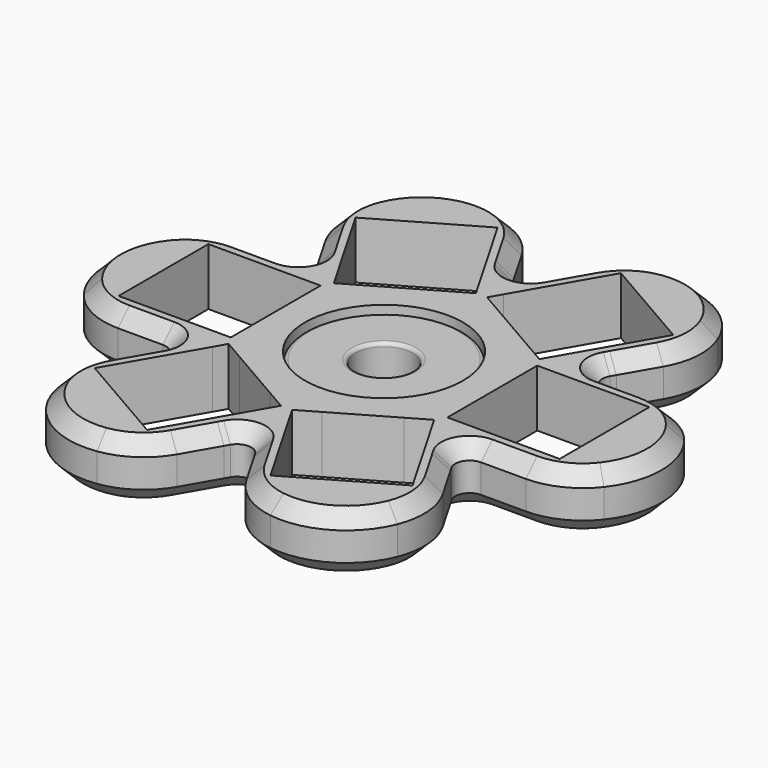
from build123d import *

# Parameters (mm, degrees)
F0_R     = 11
F0_R_2   = 4
F1_DEPTH = 7
F2_R     = 11.05
F3_DEPTH = 8
F4_R     = 2
F5_R     = 10
F6_SIZE  = 2
F7_R     = 0.5


# Not quite as in the source:
# - a feature names something its author has since deleted; it is built from what else it names


with BuildPart() as f1:
    # F0 (on Top) → F1 (new body)
    with BuildSketch(Plane.XY):
        Circle(F0_R)
        Circle(F0_R_2, mode=Mode.SUBTRACT)
    extrude(amount=F1_DEPTH)

    # F7
    f7_edges = [f1.edges().sort_by_distance(p)[0] for p in [
        (-11, 0, 0),
        (-4, 0, 0),
        (-11, 0, 7),
        (-4, 0, 7),
    ]]
    fillet(f7_edges, radius=F7_R)


with BuildPart() as f3:
    # F2 (on face) → F3 (new body)
    with BuildSketch(Plane(origin=(0, 0, 0), x_dir=(1, 0, 0), z_dir=(0, 0, -1))):
        with BuildLine():
            Line((18.7927512621, -10.85), (15.328649647, -10.85))
            Line((15.328649647, -10.85), (22.2232994197, -22.7918837067))
            Line((22.2232994197, -22.7918837067), (8.6267005803, -30.6418837067))
            Line((8.6267005803, -30.6418837067), (1.7320508076, -18.7))
            Line((1.7320508076, -18.7), (0, -21.7))
            Line((0, -21.7), (2.1036243689, -25.343584287))
            Line((2.1036243689, -25.343584287), (6.0286243689, -32.1418837067))
            ThreePointArc((6.0286243689, -32.1418837067), (19.4, -33.6017856668), (24.8213756311, -21.2918837067))
            Line((24.8213756311, -21.2918837067), (20.8963756311, -14.493584287))
            Line((20.8963756311, -14.493584287), (18.7927512621, -10.85))
        make_face()
        with BuildLine():
            Line((15.15, -4.5405697347), (14.6112581801, -3.6074415304))
            ThreePointArc((14.6112581801, -3.6074415304), (13.033682327, -7.525), (10.429765098, -10.85))
            Line((10.429765098, -10.85), (11.5072487379, -10.85))
            Line((11.5072487379, -10.85), (14.3732994197, -9.1952848673))
            Line((14.3732994197, -9.1952848673), (15.328649647, -10.85))
            Line((15.328649647, -10.85), (18.7927512621, -10.85))
            Line((18.7927512621, -10.85), (17.0607004546, -7.85))
            Line((17.0607004546, -7.85), (15.15, -7.85))
            Line((15.15, -7.85), (15.15, -4.5405697347))
        make_face()
        with BuildLine():
            ThreePointArc((14.6112581801, -3.6074415304), (14.9399119075, -1.8170118863), (15.05, 0))
            ThreePointArc((15.05, 0), (14.9399119075, 1.8170118863), (14.6112581801, 3.6074415304))
            ThreePointArc((14.6112581801, 3.6074415304), (13.033682327, 7.525), (10.429765098, 10.85))
            ThreePointArc((10.429765098, 10.85), (7.525, 13.033682327), (4.181493082, 14.4574415304))
            ThreePointArc((4.181493082, 14.4574415304), (0, 15.05), (-4.181493082, 14.4574415304))
            ThreePointArc((-4.181493082, 14.4574415304), (-7.525, 13.033682327), (-10.429765098, 10.85))
            ThreePointArc((-10.429765098, 10.85), (-13.033682327, 7.525), (-14.6112581801, 3.6074415304))
            ThreePointArc((-14.6112581801, 3.6074415304), (-15.05, 0), (-14.6112581801, -3.6074415304))
            ThreePointArc((-14.6112581801, -3.6074415304), (-13.033682327, -7.525), (-10.429765098, -10.85))
            ThreePointArc((-10.429765098, -10.85), (-7.525, -13.033682327), (-4.181493082, -14.4574415304))
            ThreePointArc((-4.181493082, -14.4574415304), (0, -15.05), (4.181493082, -14.4574415304))
            ThreePointArc((4.181493082, -14.4574415304), (7.525, -13.033682327), (10.429765098, -10.85))
            ThreePointArc((10.429765098, -10.85), (13.033682327, -7.525), (14.6112581801, -3.6074415304))
        make_face()
        Circle(F2_R, mode=Mode.SUBTRACT)
        with BuildLine():
            Line((0, -21.7), (-1.7320508076, -18.7))
            Line((-1.7320508076, -18.7), (-8.6267005803, -30.6418837067))
            Line((-8.6267005803, -30.6418837067), (-22.2232994197, -22.7918837067))
            Line((-22.2232994197, -22.7918837067), (-15.328649647, -10.85))
            Line((-15.328649647, -10.85), (-18.7927512621, -10.85))
            Line((-18.7927512621, -10.85), (-20.8963756311, -14.493584287))
            Line((-20.8963756311, -14.493584287), (-24.8213756311, -21.2918837067))
            ThreePointArc((-24.8213756311, -21.2918837067), (-19.4, -33.6017856668), (-6.0286243689, -32.1418837067))
            Line((-6.0286243689, -32.1418837067), (-2.1036243689, -25.343584287))
            Line((-2.1036243689, -25.343584287), (0, -21.7))
        make_face()
        with BuildLine():
            Line((3.6427512621, -15.3905697347), (4.181493082, -14.4574415304))
            ThreePointArc((4.181493082, -14.4574415304), (0, -15.05), (-4.181493082, -14.4574415304))
            Line((-4.181493082, -14.4574415304), (-3.6427512621, -15.3905697347))
            Line((-3.6427512621, -15.3905697347), (-0.7767005803, -17.0452848673))
            Line((-0.7767005803, -17.0452848673), (-1.7320508076, -18.7))
            Line((-1.7320508076, -18.7), (0, -21.7))
            Line((0, -21.7), (1.7320508076, -18.7))
            Line((1.7320508076, -18.7), (0.7767005803, -17.0452848673))
            Line((0.7767005803, -17.0452848673), (3.6427512621, -15.3905697347))
        make_face()
        with BuildLine():
            Line((-30.85, 7.85), (-17.0607004546, 7.85))
            Line((-17.0607004546, 7.85), (-18.7927512621, 10.85))
            Line((-18.7927512621, 10.85), (-23, 10.85))
            Line((-23, 10.85), (-30.85, 10.85))
            ThreePointArc((-30.85, 10.85), (-38.8, 0), (-30.85, -10.85))
            Line((-30.85, -10.85), (-23, -10.85))
            Line((-23, -10.85), (-18.7927512621, -10.85))
            Line((-18.7927512621, -10.85), (-17.0607004546, -7.85))
            Line((-17.0607004546, -7.85), (-30.85, -7.85))
            Line((-30.85, -7.85), (-30.85, 7.85))
        make_face()
        with BuildLine():
            Line((-11.5072487379, -10.85), (-10.429765098, -10.85))
            ThreePointArc((-10.429765098, -10.85), (-13.033682327, -7.525), (-14.6112581801, -3.6074415304))
            Line((-14.6112581801, -3.6074415304), (-15.15, -4.5405697347))
            Line((-15.15, -4.5405697347), (-15.15, -7.85))
            Line((-15.15, -7.85), (-17.0607004546, -7.85))
            Line((-17.0607004546, -7.85), (-18.7927512621, -10.85))
            Line((-18.7927512621, -10.85), (-15.328649647, -10.85))
            Line((-15.328649647, -10.85), (-14.3732994197, -9.1952848673))
            Line((-14.3732994197, -9.1952848673), (-11.5072487379, -10.85))
        make_face()
        with BuildLine():
            Line((18.7927512621, 10.85), (17.0607004546, 7.85))
            Line((17.0607004546, 7.85), (30.85, 7.85))
            Line((30.85, 7.85), (30.85, -7.85))
            Line((30.85, -7.85), (17.0607004546, -7.85))
            Line((17.0607004546, -7.85), (18.7927512621, -10.85))
            Line((18.7927512621, -10.85), (23, -10.85))
            Line((23, -10.85), (30.85, -10.85))
            ThreePointArc((30.85, -10.85), (38.8, 0), (30.85, 10.85))
            Line((30.85, 10.85), (23, 10.85))
            Line((23, 10.85), (18.7927512621, 10.85))
        make_face()
        with BuildLine():
            Line((22.2232994197, 22.7918837067), (15.328649647, 10.85))
            Line((15.328649647, 10.85), (18.7927512621, 10.85))
            Line((18.7927512621, 10.85), (20.8963756311, 14.493584287))
            Line((20.8963756311, 14.493584287), (24.8213756311, 21.2918837067))
            ThreePointArc((24.8213756311, 21.2918837067), (19.4, 33.6017856668), (6.0286243689, 32.1418837067))
            Line((6.0286243689, 32.1418837067), (2.1036243689, 25.343584287))
            Line((2.1036243689, 25.343584287), (0, 21.7))
            Line((0, 21.7), (1.7320508076, 18.7))
            Line((1.7320508076, 18.7), (8.6267005803, 30.6418837067))
            Line((8.6267005803, 30.6418837067), (22.2232994197, 22.7918837067))
        make_face()
        with BuildLine():
            Line((-8.6267005803, 30.6418837067), (-1.7320508076, 18.7))
            Line((-1.7320508076, 18.7), (0, 21.7))
            Line((0, 21.7), (-2.1036243689, 25.343584287))
            Line((-2.1036243689, 25.343584287), (-6.0286243689, 32.1418837067))
            ThreePointArc((-6.0286243689, 32.1418837067), (-19.4, 33.6017856668), (-24.8213756311, 21.2918837067))
            Line((-24.8213756311, 21.2918837067), (-20.8963756311, 14.493584287))
            Line((-20.8963756311, 14.493584287), (-18.7927512621, 10.85))
            Line((-18.7927512621, 10.85), (-15.328649647, 10.85))
            Line((-15.328649647, 10.85), (-22.2232994197, 22.7918837067))
            Line((-22.2232994197, 22.7918837067), (-8.6267005803, 30.6418837067))
        make_face()
        with BuildLine():
            ThreePointArc((-4.181493082, 14.4574415304), (0, 15.05), (4.181493082, 14.4574415304))
            Line((4.181493082, 14.4574415304), (3.6427512621, 15.3905697347))
            Line((3.6427512621, 15.3905697347), (0.7767005803, 17.0452848673))
            Line((0.7767005803, 17.0452848673), (1.7320508076, 18.7))
            Line((1.7320508076, 18.7), (0, 21.7))
            Line((0, 21.7), (-1.7320508076, 18.7))
            Line((-1.7320508076, 18.7), (-0.7767005803, 17.0452848673))
            Line((-0.7767005803, 17.0452848673), (-3.6427512621, 15.3905697347))
            Line((-3.6427512621, 15.3905697347), (-4.181493082, 14.4574415304))
        make_face()
        with BuildLine():
            ThreePointArc((10.429765098, 10.85), (13.033682327, 7.525), (14.6112581801, 3.6074415304))
            Line((14.6112581801, 3.6074415304), (15.15, 4.5405697347))
            Line((15.15, 4.5405697347), (15.15, 7.85))
            Line((15.15, 7.85), (17.0607004546, 7.85))
            Line((17.0607004546, 7.85), (18.7927512621, 10.85))
            Line((18.7927512621, 10.85), (15.328649647, 10.85))
            Line((15.328649647, 10.85), (14.3732994197, 9.1952848673))
            Line((14.3732994197, 9.1952848673), (11.5072487379, 10.85))
            Line((11.5072487379, 10.85), (10.429765098, 10.85))
        make_face()
        with BuildLine():
            ThreePointArc((-14.6112581801, 3.6074415304), (-13.033682327, 7.525), (-10.429765098, 10.85))
            Line((-10.429765098, 10.85), (-11.5072487379, 10.85))
            Line((-11.5072487379, 10.85), (-14.3732994197, 9.1952848673))
            Line((-14.3732994197, 9.1952848673), (-15.328649647, 10.85))
            Line((-15.328649647, 10.85), (-18.7927512621, 10.85))
            Line((-18.7927512621, 10.85), (-17.0607004546, 7.85))
            Line((-17.0607004546, 7.85), (-15.15, 7.85))
            Line((-15.15, 7.85), (-15.15, 4.5405697347))
            Line((-15.15, 4.5405697347), (-14.6112581801, 3.6074415304))
        make_face()
        with BuildLine():
            ThreePointArc((-10.429765098, 10.85), (-7.525, 13.033682327), (-4.181493082, 14.4574415304))
            Line((-4.181493082, 14.4574415304), (-3.6427512621, 15.3905697347))
            Line((-3.6427512621, 15.3905697347), (-11.5072487379, 10.85))
            Line((-11.5072487379, 10.85), (-10.429765098, 10.85))
        make_face()
        with BuildLine():
            ThreePointArc((4.181493082, 14.4574415304), (7.525, 13.033682327), (10.429765098, 10.85))
            Line((10.429765098, 10.85), (11.5072487379, 10.85))
            Line((11.5072487379, 10.85), (3.6427512621, 15.3905697347))
            Line((3.6427512621, 15.3905697347), (4.181493082, 14.4574415304))
        make_face()
        with BuildLine():
            ThreePointArc((14.6112581801, 3.6074415304), (14.9399119075, 1.8170118863), (15.05, 0))
            ThreePointArc((15.05, 0), (14.9399119075, -1.8170118863), (14.6112581801, -3.6074415304))
            Line((14.6112581801, -3.6074415304), (15.15, -4.5405697347))
            Line((15.15, -4.5405697347), (15.15, 4.5405697347))
            Line((15.15, 4.5405697347), (14.6112581801, 3.6074415304))
        make_face()
        with BuildLine():
            Line((11.5072487379, -10.85), (10.429765098, -10.85))
            ThreePointArc((10.429765098, -10.85), (7.525, -13.033682327), (4.181493082, -14.4574415304))
            Line((4.181493082, -14.4574415304), (3.6427512621, -15.3905697347))
            Line((3.6427512621, -15.3905697347), (11.5072487379, -10.85))
        make_face()
        with BuildLine():
            Line((-3.6427512621, -15.3905697347), (-4.181493082, -14.4574415304))
            ThreePointArc((-4.181493082, -14.4574415304), (-7.525, -13.033682327), (-10.429765098, -10.85))
            Line((-10.429765098, -10.85), (-11.5072487379, -10.85))
            Line((-11.5072487379, -10.85), (-3.6427512621, -15.3905697347))
        make_face()
        with BuildLine():
            ThreePointArc((-14.6112581801, -3.6074415304), (-15.05, 0), (-14.6112581801, 3.6074415304))
            Line((-14.6112581801, 3.6074415304), (-15.15, 4.5405697347))
            Line((-15.15, 4.5405697347), (-15.15, -4.5405697347))
            Line((-15.15, -4.5405697347), (-14.6112581801, -3.6074415304))
        make_face()
    extrude(amount=-F3_DEPTH)

    # F4
    f4_edges = [f3.edges().sort_by_distance(p)[0] for p in [
        (-18.792751, 10.85, 4),
        (0, 21.7, 4),
        (18.792751, 10.85, 4),
        (0, -21.7, 4),
        (-18.792751, -10.85, 4),
        (18.792751, -10.85, 4),
    ]]
    fillet(f4_edges, radius=F4_R)

    # F5
    f5_edges = [f3.edges().sort_by_distance(p)[0] for p in [
        (24.821376, -21.291884, 4),
        (30.85, -10.85, 4),
        (30.85, 10.85, 4),
        (24.821376, 21.291884, 4),
        (6.028624, 32.141884, 4),
        (-6.028624, 32.141884, 4),
        (-24.821376, 21.291884, 4),
        (-30.85, 10.85, 4),
        (-30.85, -10.85, 4),
        (-24.821376, -21.291884, 4),
        (-6.028624, -32.141884, 4),
        (6.028624, -32.141884, 4),
    ]]
    fillet(f5_edges, radius=F5_R)

    # F6
    f6_edges = [f3.edges().sort_by_distance(p)[0] for p in [
        (19.4, 33.601786, 8),
        (-19.4, 33.601786, 8),
        (-32.88625, -9.840049, 8),
        (19.4, 33.601786, 0),
        (-38.8, 0, 0),
        (-19.4, 33.601786, 0),
    ]]
    chamfer(f6_edges, length=F6_SIZE)


solid = Compound([f1.part, f3.part])
